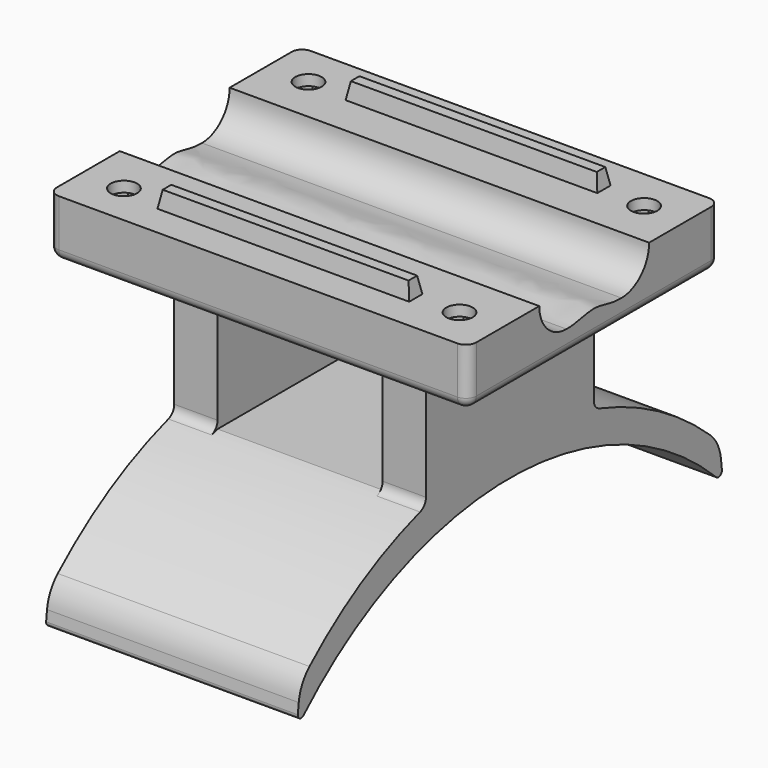
from build123d import *

# Parameters (mm, degrees)
F1_W          = 50.8
F1_H          = 38.1
F2_DEPTH      = 6.985
F4_DEPTH      = 50.8
F6_DEPTH      = 15.24
F6_DEPTH_BACK = 15.24
F7_W          = 20
F7_H          = 15.8292923384
F8_DEPTH      = 25.4
F9_R          = 1.6
F10_DEPTH     = 25.4
F11_R         = 1.6
F12_DEPTH     = 5.7
F13_W         = 30.48
F13_H         = 2
F14_DEPTH     = 2
F14_TAPER     = 10
F15_R         = 0.508
F16_R         = 5.08
F17_R         = 1.27


# Not quite as in the source:
# - two fillets or chamfers of one size are made in one step


with BuildPart() as f2:
    # F1 (on Top) → F2 (new body)
    with BuildSketch(Plane.XY):
        Rectangle(F1_W, F1_H)
    extrude(amount=-F2_DEPTH)

    # F3 (on face) → F4 (cut, through all)
    with BuildSketch(Plane.YZ.offset(25.4)):
        with BuildLine():
            add(Edge.make_bspline(
                [(-4.125, 4.125), (-2.4255892558, 4.1137489608), (-0.0276085061, 2.971292738), (2.5249406681, 4.1137612248), (4.191, 4.191)],
                knots=[0, 0, 0, 0, 0.4977710734, 1, 1, 1, 1], degree=3))
            ThreePointArc((-4.125, 4.125), (-7.0418154724, 2.9168154724), (-8.25, 0))
            ThreePointArc((-8.25, 0), (-7.0418154724, -2.9168154724), (-4.125, -4.125))
            add(Edge.make_bspline(
                [(-4.125, -4.125), (-2.9335741419, -4.2006121948), (0.4172014685, -3.0581585459), (2.1438994445, -4.2006121948), (4.191, -4.191)],
                knots=[0, 0, 0, 0, 0.497799261, 1, 1, 1, 1], degree=3))
            ThreePointArc((4.191, -4.191), (7.15448452, -2.96348452), (8.382, 0))
            ThreePointArc((8.382, 0), (7.15448452, 2.96348452), (4.191, 4.191))
        make_face()
    extrude(amount=-F4_DEPTH, mode=Mode.SUBTRACT)

    # F5 (on Right) → F6 (join, two sides)
    with BuildSketch(Plane.YZ) as f6_sk:
        with BuildLine():
            ThreePointArc((-32.258, -38.6095089919), (0, -24.985), (32.258, -38.6095089919))
            Line((32.258, -38.6095089919), (31.75, -34.0955424944))
            ThreePointArc((31.75, -34.0955424944), (22.9296157026, -27.265073299), (12.7, -22.8142923384))
            ThreePointArc((12.7, -22.8142923384), (0, -20.985), (-12.7, -22.8142923384))
            ThreePointArc((-12.7, -22.8142923384), (-22.9296157026, -27.265073299), (-31.75, -34.0955424944))
            Line((-31.75, -34.0955424944), (-32.258, -38.6095089919))
        make_face()
        with BuildLine():
            ThreePointArc((-12.7, -22.8142923384), (0, -20.985), (12.7, -22.8142923384))
            Line((12.7, -22.8142923384), (12.7, -6.985))
            Line((12.7, -6.985), (-12.7, -6.985))
            Line((-12.7, -6.985), (-12.7, -22.8142923384))
        make_face()
    extrude(amount=F6_DEPTH)
    extrude(f6_sk.sketch, amount=-F6_DEPTH_BACK)

    # F7 (on face) → F8 (cut)
    with BuildSketch(Plane.XZ.offset(12.7)):
        with Locations((0, -14.8996461692)):
            Rectangle(F7_W, F7_H)
    extrude(amount=-F8_DEPTH, mode=Mode.SUBTRACT)

    # F9 (on face) → F10 (cut)
    with BuildSketch(Plane(origin=(0, 0, -6.985), x_dir=(1, 0, 0), z_dir=(0, 0, -1))):
        with Locations((20.32, -13.97)):
            Circle(F9_R)
        with Locations((-20.32, -13.97)):
            Circle(F9_R)
        with Locations((-20.32, 13.97)):
            Circle(F9_R)
        with Locations((20.32, 13.97)):
            Circle(F9_R)
    extrude(amount=-F10_DEPTH, mode=Mode.SUBTRACT)

    # F11 (on face) → F12 (cut)
    with BuildSketch(Plane(origin=(0, 0, -6.985), x_dir=(1, 0, 0), z_dir=(0, 0, -1))):
        Polygon((21.645, -16.26496732), (22.97, -13.97), (21.645, -11.67503268), (18.995, -11.67503268), (17.67, -13.97), (18.995, -16.26496732), align=None)
        with Locations((20.32, -13.97)):
            Circle(F11_R, mode=Mode.SUBTRACT)
        Polygon((-18.995, -11.67503268), (-21.645, -11.67503268), (-22.97, -13.97), (-21.645, -16.26496732), (-18.995, -16.26496732), (-17.67, -13.97), align=None)
        with Locations((-20.32, -13.97)):
            Circle(F11_R, mode=Mode.SUBTRACT)
        Polygon((-18.995, 11.67503268), (-17.67, 13.97), (-18.995, 16.26496732), (-21.645, 16.26496732), (-22.97, 13.97), (-21.645, 11.67503268), align=None)
        with Locations((-20.32, 13.97)):
            Circle(F11_R, mode=Mode.SUBTRACT)
        Polygon((18.995, 11.67503268), (21.645, 11.67503268), (22.97, 13.97), (21.645, 16.26496732), (18.995, 16.26496732), (17.67, 13.97), align=None)
        with Locations((20.32, 13.97)):
            Circle(F11_R, mode=Mode.SUBTRACT)
    extrude(amount=-F12_DEPTH, mode=Mode.SUBTRACT)

    # F13 (on face) → F14 (join)
    with BuildSketch(Plane.XY):
        with Locations((0, 14.24)):
            Rectangle(F13_W, F13_H)
        with Locations((0, -14.24)):
            Rectangle(F13_W, F13_H)
    extrude(amount=F14_DEPTH, taper=F14_TAPER)

    # F15
    f15_edges = [f2.edges().sort_by_distance(p)[0] for p in [
        (0, 32.258, -38.609509),
        (0, -32.258, -38.609509),
    ]]
    fillet(f15_edges, radius=F15_R)

    # F16
    f16_edges = [f2.edges().sort_by_distance(p)[0] for p in [
        (0, 31.75, -34.095542),
        (0, -31.75, -34.095542),
    ]]
    fillet(f16_edges, radius=F16_R)

    # F17
    f17_edges = [f2.edges().sort_by_distance(p)[0] for p in [
        (-15.24, 0, -6.985),
        (12.62, -12.7, -22.814292),
        (-12.62, -12.7, -22.814292),
        (-12.62, -12.7, -6.985),
        (0, 19.05, -6.985),
        (25.4, 0, -6.985),
        (-25.4, 0, -6.985),
        (0, -19.05, -6.985),
        (-12.62, 12.7, -6.985),
        (-10, 0, -6.985),
        (12.62, -12.7, -6.985),
        (10, 0, -6.985),
        (15.24, 0, -6.985),
        (12.62, 12.7, -6.985),
        (-12.62, 12.7, -22.814292),
        (12.62, 12.7, -22.814292),
        (25.4, 19.05, -3.4925),
        (-25.4, 19.05, -3.4925),
        (25.4, -19.05, -3.4925),
        (-25.4, -19.05, -3.4925),
    ]]
    fillet(f17_edges, radius=F17_R)


solid = f2.part
